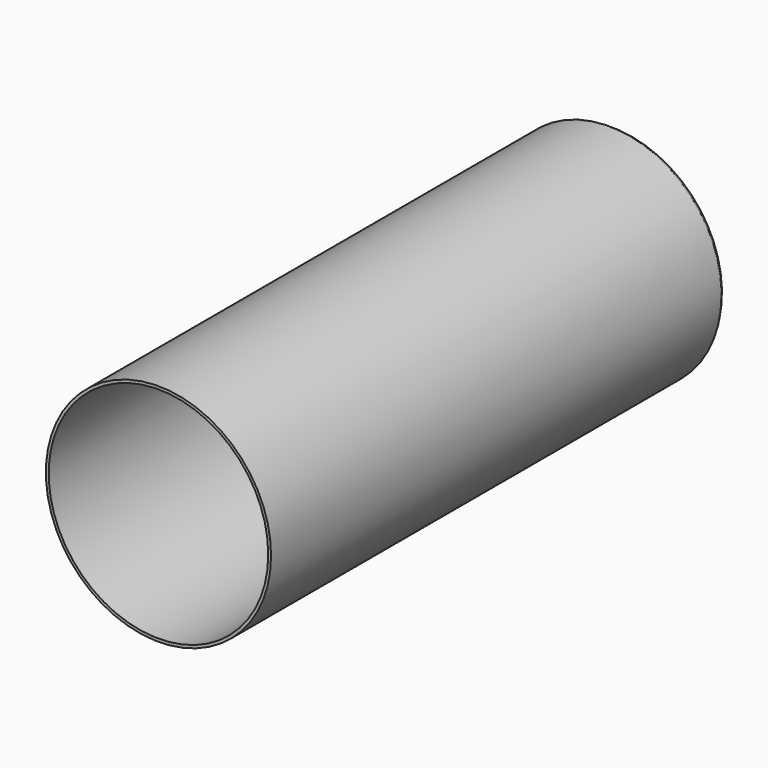
from build123d import *

# Parameters (mm, degrees)
F0_R     = 40
F0_R_2   = 39
F1_DEPTH = 200


# Not quite as in the source:
# - a fillet or chamfer that OpenCascade refuses, or shapes differently, is made with other operations: its cross-section is extruded or revolved along the edge and cut away or added


with BuildPart() as f1:
    # F0 (on Front) → F1 (new body)
    with BuildSketch(Plane.XZ):
        Circle(F0_R)
        Circle(F0_R_2, mode=Mode.SUBTRACT)
    extrude(amount=F1_DEPTH)

    # F2 (on Right) → F3 (revolve)
    with BuildSketch(Plane.YZ):
        Polygon((0, 0), (0, -39.8333705962), (3, -39.8333705962), (6, 0), align=None)
    revolve(axis=Axis((0, 3, 0), (0, -1, 0)))

    # F4: fillet of radius 5 on 1 edges, made by hand

    # F4_s1 → F4_t2 (revolve, cut)
    with BuildSketch(Plane.YZ):
        with BuildLine():
            ThreePointArc((0.000132768, -39.8337479192), (2.3100716804, -38.1578030018), (3.3274101289, -35.4914137529))
            Line((3.3274101289, -35.4914137529), (3.8261475828, -35.5289755344))
            ThreePointArc((3.8261475828, -35.5289755344), (3.6622430832, -37.6999389358), (3.4987374539, -39.8709323776))
            Line((3.4987374539, -39.8709323776), (3, -40.3335205091))
            ThreePointArc((3, -40.3335205091), (1.500066384, -40.3335205091), (0.1661424858, -40.3055431173))
            Line((0.1661424858, -40.3055431173), (0.000132768, -39.8337479192))
        make_face()
    revolve(axis=Axis((0, 3, 0), (0, -1, 0)), mode=Mode.SUBTRACT)


solid = f1.part
